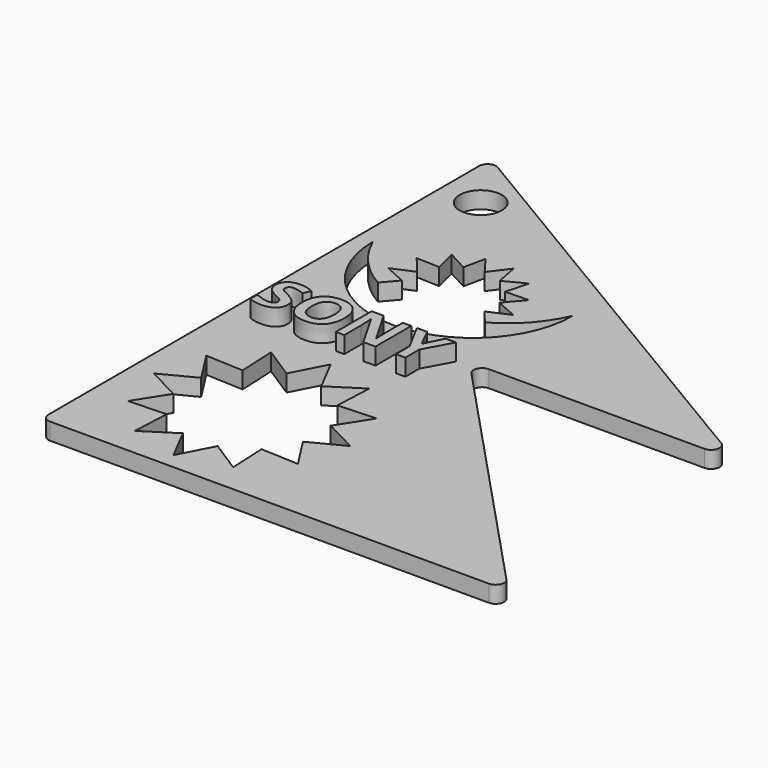
from build123d import *

# Parameters (mm, degrees)
F2_DEPTH     = 2
F3_DEPTH     = 25
F4_R         = 1
F5_TEXT_SIZE = 7.4370692213
F6_DEPTH     = 2
F7_R         = 2.5
F8_DEPTH     = 25


# Not quite as in the source:
# - Text() gives the source's letters only with a copy of the font that has no kerning and outlines rounded to 1/6400 em; it was checked with that copy


with BuildPart() as f2:
    # F0 (on Top) → F2 (new body)
    with BuildSketch(Plane.XY):
        Polygon((55.4308257997, 33.6407795548), (0, 66.7081326246), (0, 0), (55.4308257997, 0), (23.8926000893, 33.6407795548), align=None)
        Polygon((12.0832106018, 21.2485467089), (14.1444178298, 25.2305828035), (16.2056250578, 21.2485467089), (19.981700927, 23.6664875116), (19.7757407016, 19.1873394809), (24.2548887323, 19.3932997063), (21.8369479296, 15.6172238371), (25.8189840242, 13.5560166091), (21.8369479296, 11.4948093811), (24.2548887323, 7.7187335119), (19.7757407016, 7.9246937373), (19.981700927, 3.4455457065), (16.2056250578, 5.8634865093), (14.1444178298, 1.8814504147), (12.0832106018, 5.8634865093), (8.3071347326, 3.4455457065), (8.513094958, 7.9246937373), (4.0339469273, 7.7187335119), (6.45188773, 11.4948093811), (2.4698516354, 13.5560166091), (6.45188773, 15.6172238371), (4.0339469273, 19.3932997063), (8.513094958, 19.1873394809), (8.3071347326, 23.6664875116), align=None, mode=Mode.SUBTRACT)
    extrude(amount=-F2_DEPTH)

    # F1 (on face) → F3 (cut)
    with BuildSketch(Plane.XY):
        with BuildLine():
            ThreePointArc((7.2890369966, 40.7889018386), (4.0560250019, 43.4007835408), (1.8165675739, 46.9020865858))
            ThreePointArc((1.8165675739, 46.9020865858), (13.7077793479, 35.0108748118), (25.5989911219, 46.9020865858))
            ThreePointArc((25.5989911219, 46.9020865858), (23.3308399618, 43.3688370595), (20.0517837382, 40.7465952358))
            Line((20.0517837382, 40.7465952358), (18.6294270351, 42.4385848131))
            Line((18.6294270351, 42.4385848131), (21.1653646925, 43.5567679213))
            Line((21.1653646925, 43.5567679213), (18.6369902604, 44.6919489626))
            Line((18.6369902604, 44.6919489626), (20.4346075717, 46.8014240792))
            Line((20.4346075717, 46.8014240792), (17.6641568122, 46.7245094843))
            Line((17.6641568122, 46.7245094843), (18.3659162196, 49.405712013))
            Line((18.3659162196, 49.405712013), (15.9044186498, 48.1319997301))
            Line((15.9044186498, 48.1319997301), (15.3707435352, 50.8516512037))
            Line((15.3707435352, 50.8516512037), (13.7077793479, 48.6344765652))
            Line((13.7077793479, 48.6344765652), (12.1176077334, 50.7545992963))
            Line((12.1176077334, 50.7545992963), (11.5724253998, 48.1610799921))
            Line((11.5724253998, 48.1610799921), (9.1282495157, 49.467723598))
            Line((9.1282495157, 49.467723598), (9.7939499818, 46.7773414402))
            Line((9.7939499818, 46.7773414402), (7.0247814956, 46.8914429764))
            Line((7.0247814956, 46.8914429764), (8.7939166631, 44.7580245869))
            Line((8.7939166631, 44.7580245869), (6.2505300539, 43.656889799))
            Line((6.2505300539, 43.656889799), (8.7712273282, 42.5047619776))
            Line((8.7712273282, 42.5047619776), (7.2890369966, 40.7889018386))
        make_face()
    extrude(amount=-F3_DEPTH, mode=Mode.SUBTRACT)

    # F4
    f4_edges = [f2.edges().sort_by_distance(p)[0] for p in [
        (0, 0, -1),
        (55.430826, 0, -1),
        (23.8926, 33.64078, -1),
        (55.430826, 33.64078, -1),
        (0, 66.708133, -1),
    ]]
    fillet(f4_edges, radius=F4_R)

    # F5 (on face) → F6 (join)
    with BuildSketch(Plane.XY):
        with Locations((2.1602446274, 27.6188906282)):
            Text('SONY', F5_TEXT_SIZE, font='Open Sans', font_style=FontStyle.BOLD, text_align=(TextAlign.LEFT, TextAlign.BOTTOM))
    extrude(amount=F6_DEPTH)

    # F7 (on face) → F8 (cut)
    with BuildSketch(Plane.XY):
        with Locations((4.7155795619, 59.2868067324)):
            Circle(F7_R)
    extrude(amount=-F8_DEPTH, mode=Mode.SUBTRACT)


solid = f2.part
